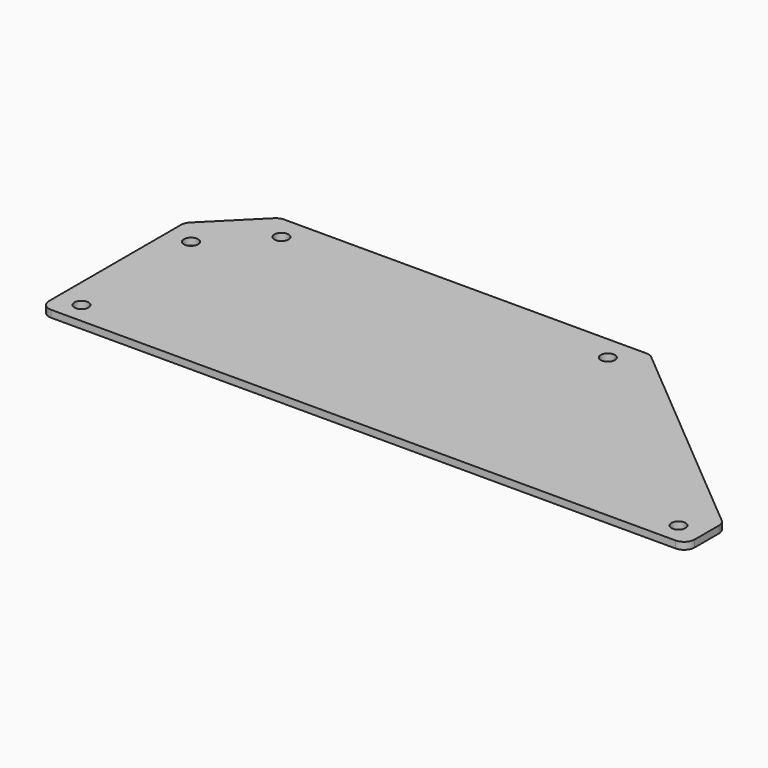
from build123d import *

# Parameters (mm, degrees)
F0_R     = 2
F1_DEPTH = 2


# Not quite as in the source:
# - ends of sketch curves that miss each other by under 0.0002 mm in the source are joined


with BuildPart() as f1:
    # F0 (on Top) → F1 (new body)
    with BuildSketch(Plane.XY):
        with BuildLine():
            ThreePointArc((91.5, -21.3966), (91.2197291677, -20.1304747082), (90.4312844969, -19.1009214093))
            Line((90.4312844969, -19.1009214093), (29.337212, 32.295678))
            ThreePointArc((29.337212, 32.295678), (28.4337805172, 32.818424586), (27.405927, 33))
            Line((27.405927, 33), (-75.25736, 33))
            ThreePointArc((-75.25736, 33), (-76.4054102971, 32.7716385975), (-77.3786803436, 32.1213203436))
            Line((-77.3786803436, 32.1213203436), (-90.621321, 18.87868))
            ThreePointArc((-90.621321, 18.87868), (-91.2716385975, 17.9054092971), (-91.5, 16.757359))
            Line((-91.5, 16.757359), (-91.5, -30))
            ThreePointArc((-91.5, -30), (-90.6213203436, -32.1213203436), (-88.5, -33))
            Line((-88.5, -33), (88.5, -33))
            ThreePointArc((88.5, -33), (90.6213203436, -32.1213203436), (91.5, -30))
            Line((91.5, -30), (91.5, -21.3966))
        make_face()
        with Locations((-84.7, -27)):
            Circle(F0_R, mode=Mode.SUBTRACT)
        with Locations((84.5, -27)):
            Circle(F0_R, mode=Mode.SUBTRACT)
        with Locations((-84.7, 11.8)):
            Circle(F0_R, mode=Mode.SUBTRACT)
        with Locations((-70.5, 26.1)):
            Circle(F0_R, mode=Mode.SUBTRACT)
        with Locations((22, 26.1)):
            Circle(F0_R, mode=Mode.SUBTRACT)
    extrude(amount=F1_DEPTH)


solid = f1.part
